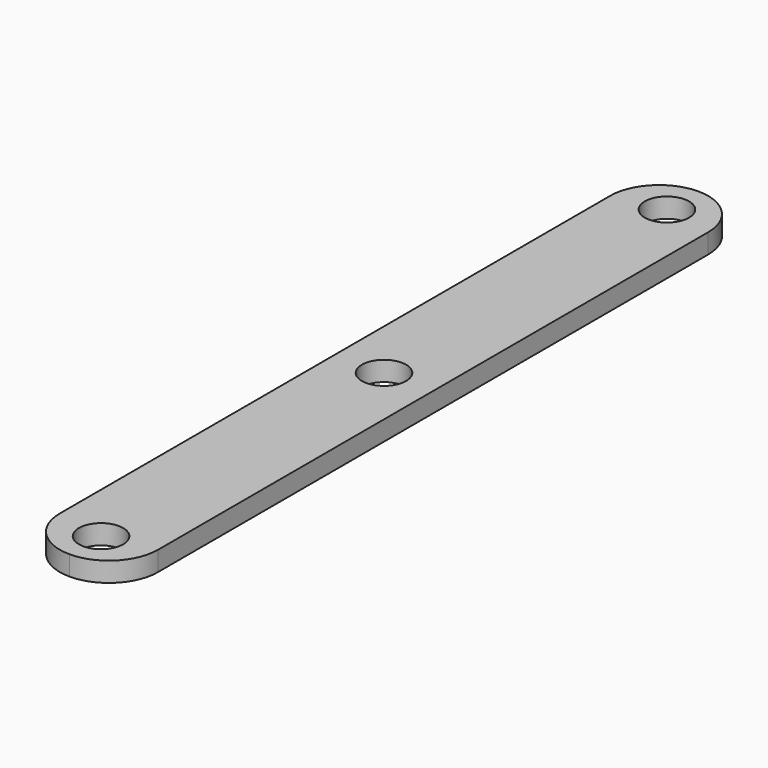
from build123d import *

# Parameters (mm, degrees)
F0_W     = 12.7
F0_H     = 101.6
F0_R     = 2.8575
F1_DEPTH = 2.54
F2_R     = 6.34999


# Not quite as in the source:
# - a fillet or chamfer is up to 0.001 mm smaller than in the source, because OpenCascade refuses the exact size


with BuildPart() as f1:
    # F0 (on Top) → F1 (new body)
    with BuildSketch(Plane.XY):
        Rectangle(F0_W, F0_H)
        with Locations((0, -45.72)):
            Circle(F0_R, mode=Mode.SUBTRACT)
        Circle(F0_R, mode=Mode.SUBTRACT)
        with Locations((0, 45.72)):
            Circle(F0_R, mode=Mode.SUBTRACT)
    extrude(amount=F1_DEPTH)

    # F2 (radius 6.35 in the source; OpenCascade refuses exactly that, so slightly less here)
    f2_edges = [f1.edges().sort_by_distance(p)[0] for p in [
        (6.35, -50.8, 1.27),
        (-6.35, -50.8, 1.27),
        (6.35, 50.8, 1.27),
        (-6.35, 50.8, 1.27),
    ]]
    fillet(f2_edges, radius=F2_R)


solid = f1.part
